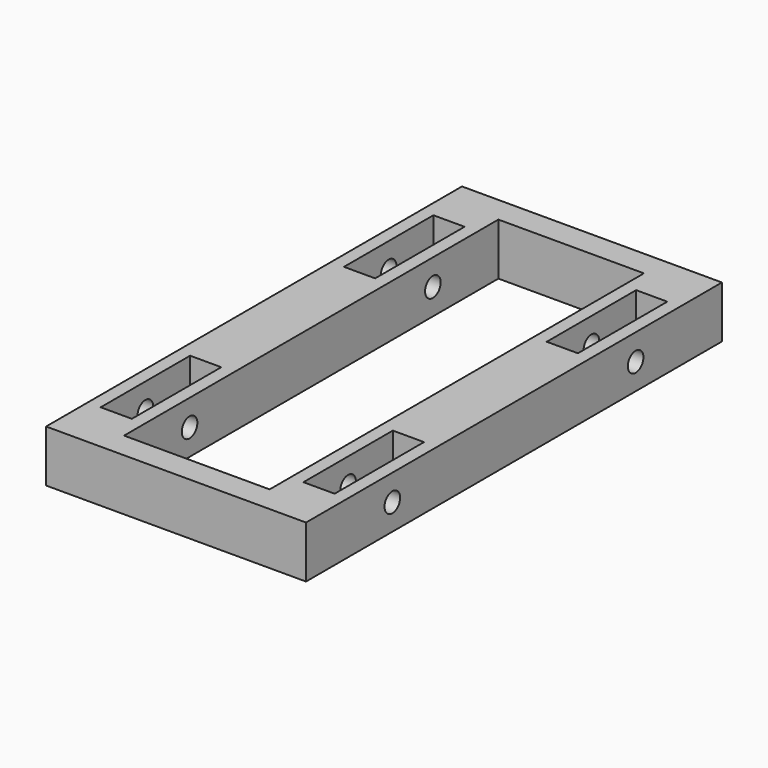
from build123d import *

# Parameters (mm, degrees)
F0_W        = 100
F0_H        = 200
F0_W_2      = 12
F0_H_2      = 43
F0_W_3      = 56
F0_H_3      = 180
F1_DEPTH    = 20
F2_R        = 3.75
F3_DEPTH    = 100.001
F4_T        = 2.5
F4_T3_DEPTH = 25


# Not quite as in the source:
# - a shell that OpenCascade refuses in one call is made with other operations: the cavity is built on its own and cut out


with BuildPart() as f1:
    # F0 (on Top) → F1 (new body)
    with BuildSketch(Plane.XY):
        with Locations((50, 100)):
            Rectangle(F0_W, F0_H)
        with Locations((11, 41.5)):
            Rectangle(F0_W_2, F0_H_2, mode=Mode.SUBTRACT)
        Polygon((89, 20), (83, 20), (83, 63), (95, 63), (95, 20), align=None, mode=Mode.SUBTRACT)
        with Locations((11, 158.5)):
            Rectangle(F0_W_2, F0_H_2, mode=Mode.SUBTRACT)
        with Locations((50, 100)):
            Rectangle(F0_W_3, F0_H_3, mode=Mode.SUBTRACT)
        with Locations((89, 158.5)):
            Rectangle(F0_W_2, F0_H_2, mode=Mode.SUBTRACT)
    extrude(amount=F1_DEPTH)

    # F2 (on face) → F3 (cut, through all)
    with BuildSketch(Plane.YZ.offset(100)):
        with Locations((41.5, 10)):
            Circle(F2_R)
        with Locations((158.5, 10)):
            Circle(F2_R)
    extrude(amount=-F3_DEPTH, mode=Mode.SUBTRACT)

    # F4: shell of thickness 2.5, made by hand


with BuildPart() as f4_core1:
    # F4_t2: copy of F1
    add(f1.part)

    # the walls: a layer under each face that stays
    f4_faces = [f4_core1.faces().sort_by_distance(p)[0] for p in [
        (0, 100, 10),
        (50, 200, 10),
        (16.6666666667, 100, 20),
        (50, 0, 10),
        (2.5, 154.75, 10),
        (2.5, 37.75, 10),
        (100, 100, 10),
        (17, 55.8333333333, 16.6666666667),
        (11, 20, 10),
        (5, 27.1666666667, 16.6666666667),
        (11, 63, 10),
        (83, 27.1666666667, 16.6666666667),
        (89, 63, 10),
        (95, 55.8333333333, 16.6666666667),
        (89, 20, 10),
        (11, 180, 10),
        (17, 172.8333333333, 16.6666666667),
        (11, 137, 10),
        (5, 144.1666666667, 16.6666666667),
        (22, 100, 10),
        (50, 190, 10),
        (78, 100, 10),
        (50, 10, 10),
        (83, 144.1666666667, 16.6666666667),
        (89, 180, 10),
        (95, 172.8333333333, 16.6666666667),
        (89, 137, 10),
        (97.5, 37.75, 10),
        (97.5, 154.75, 10),
        (19.5, 37.75, 10),
        (80.5, 37.75, 10),
        (19.5, 154.75, 10),
        (80.5, 154.75, 10),
    ]]
    thicken(f4_faces, amount=-F4_T, mode=Mode.SUBTRACT)

    # F4_s4 → F4_t3 (cut)
    with BuildSketch(Plane.XY.offset(-2.5)):
        Polygon((16.975, 62.975), (19.5, 63), (19.5, 65.5), (17, 65.5), align=None)
        Polygon((16.975, 20.025), (19.5, 20), (19.5, 17.5), (17, 17.5), align=None)
        Polygon((5.025, 20.025), (5, 17.5), (2.5, 17.5), (2.5, 20), align=None)
        Polygon((5.025, 62.975), (2.5, 63), (2.5, 65.5), (5, 65.5), align=None)
        Polygon((83.025, 20.025), (80.5, 20), (80.5, 17.5), (83, 17.5), align=None)
        Polygon((83.025, 62.975), (80.5, 63), (80.5, 65.5), (83, 65.5), align=None)
        Polygon((94.975, 62.975), (95, 65.5), (97.5, 65.5), (97.5, 63), align=None)
        Polygon((94.975, 20.025), (97.5, 20), (97.5, 17.5), (95, 17.5), align=None)
        Polygon((5.025, 179.975), (5, 182.5), (2.5, 182.5), (2.5, 180), align=None)
        Polygon((16.975, 179.975), (17, 182.5), (19.5, 182.5), (19.5, 180), align=None)
        Polygon((16.975, 137.025), (19.5, 137), (19.5, 134.5), (17, 134.5), align=None)
        Polygon((5.025, 137.025), (5, 134.5), (2.5, 134.5), (2.5, 137), align=None)
        Polygon((22.025, 10.025), (19.5, 10), (19.5, 7.5), (22, 7.5), align=None)
        Polygon((22.025, 189.975), (19.5, 190), (19.5, 192.5), (22, 192.5), align=None)
        Polygon((77.975, 189.975), (78, 192.5), (80.5, 192.5), (80.5, 190), align=None)
        Polygon((77.975, 10.025), (80.5, 10), (80.5, 7.5), (78, 7.5), align=None)
        Polygon((83.025, 137.025), (80.5, 137), (80.5, 134.5), (83, 134.5), align=None)
        Polygon((83.025, 179.975), (80.5, 180), (80.5, 182.5), (83, 182.5), align=None)
        Polygon((94.975, 179.975), (95, 182.5), (97.5, 182.5), (97.5, 180), align=None)
        Polygon((94.975, 137.025), (97.5, 137), (97.5, 134.5), (95, 134.5), align=None)
    extrude(amount=F4_T3_DEPTH, mode=Mode.SUBTRACT)


with BuildPart() as f1_1:
    add(f1.part)

    # what is left inside the walls is the cavity
    f4_cavity = [f4_core1.part.solids().sort_by_distance(p)[0] for p in [
        (50, 197.475, 11.666667),
        (2.525, 100, 11.666667),
        (50, 2.525, 11.666667),
        (80.525, 100, 11.666667),
    ]]
    add(f4_cavity, mode=Mode.SUBTRACT)


solid = f1_1.part
